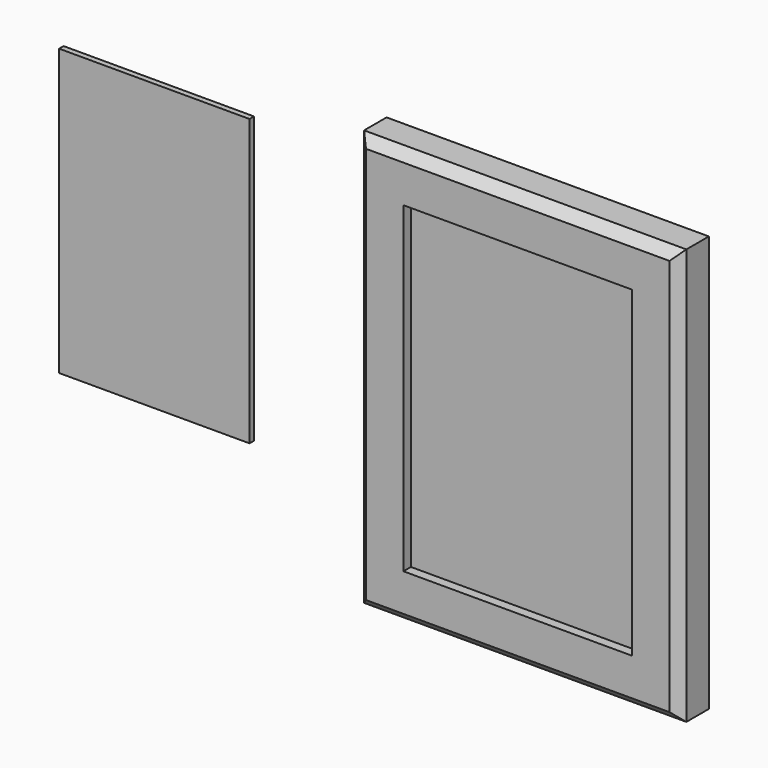
from build123d import *

# Parameters (mm, degrees)
F0_W     = 172
F0_H     = 222
F0_W_2   = 122
F0_H_2   = 172
F1_DEPTH = 20
F2_W     = 138
F2_H     = 188
F2_W_2   = 122
F2_H_2   = 172
F3_DEPTH = 15
F4_SIZE  = 5
F5_W     = 101.6
F5_H     = 152.4
F6_DEPTH = 3
F8_W     = 134
F8_H     = 184
F9_DEPTH = 3


# Not quite as in the source:
# - a feature names something its author has since deleted; it is built from what else it names


with BuildPart() as f1:
    # F0 (on Front) → F1 (new body)
    with BuildSketch(Plane.XZ):
        Rectangle(F0_W, F0_H)
        Rectangle(F0_W_2, F0_H_2, mode=Mode.SUBTRACT)
    extrude(amount=F1_DEPTH)

    # F2 (on face) → F3 (cut)
    with BuildSketch(Plane(origin=(0, 0, 0), x_dir=(-1, 0, 0), z_dir=(0, 1, 0))):
        Rectangle(F2_W, F2_H)
        Rectangle(F2_W_2, F2_H_2, mode=Mode.SUBTRACT)
    extrude(amount=-F3_DEPTH, mode=Mode.SUBTRACT)

    # F4
    f4_edges = [f1.edges().sort_by_distance(p)[0] for p in [
        (-86, -20, 0),
        (0, -20, 111),
        (86, -20, 0),
        (0, -20, -111),
    ]]
    chamfer(f4_edges, length=F4_SIZE)


with BuildPart() as f6:
    # F5 (on Front) → F6 (new body)
    with BuildSketch(Plane.XZ):
        with Locations((-207.5474485755, 12.2491330458)):
            Rectangle(F5_W, F5_H)
    extrude(amount=F6_DEPTH)


with BuildPart() as f9:
    # F8 (on face) → F9 (new body)
    with BuildSketch(Plane(origin=(0, -15, 0), x_dir=(-1, 0, 0), z_dir=(0, 1, 0))):
        Rectangle(F8_W, F8_H)
    extrude(amount=F9_DEPTH)


solid = Compound([f1.part, f6.part, f9.part])
